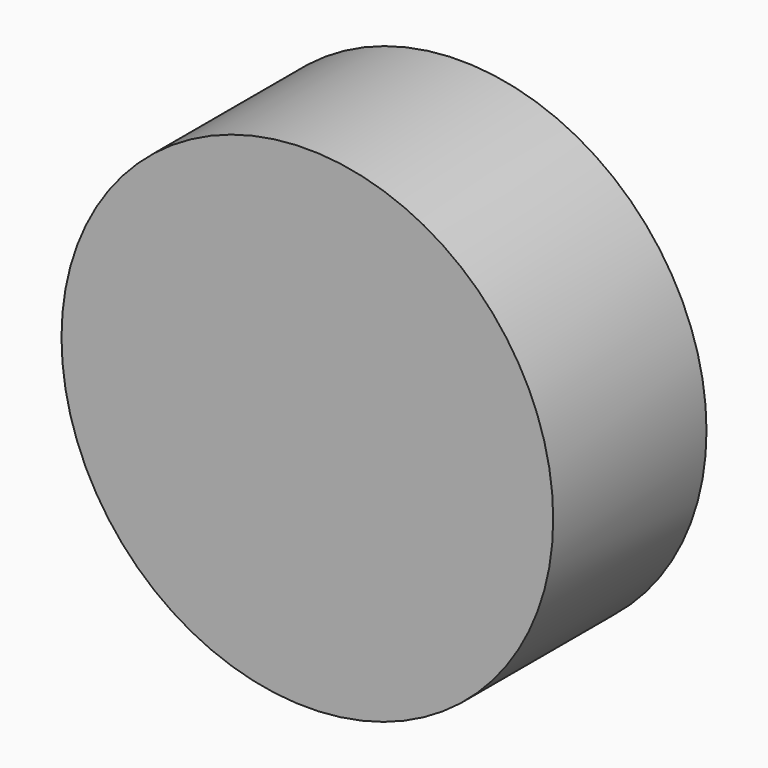
from build123d import *

# Parameters (mm, degrees)
F0_R     = 32.5900184781
F1_DEPTH = 25.4


# Not quite as in the source:
# - the program builds the solid bodies; features that only make, move or delete a surface that nothing else refers to are left out


with BuildPart() as f1:
    # F0 (on Front) → F1 (new body)
    with BuildSketch(Plane.XZ):
        Circle(F0_R)
    extrude(amount=F1_DEPTH)


solid = f1.part
